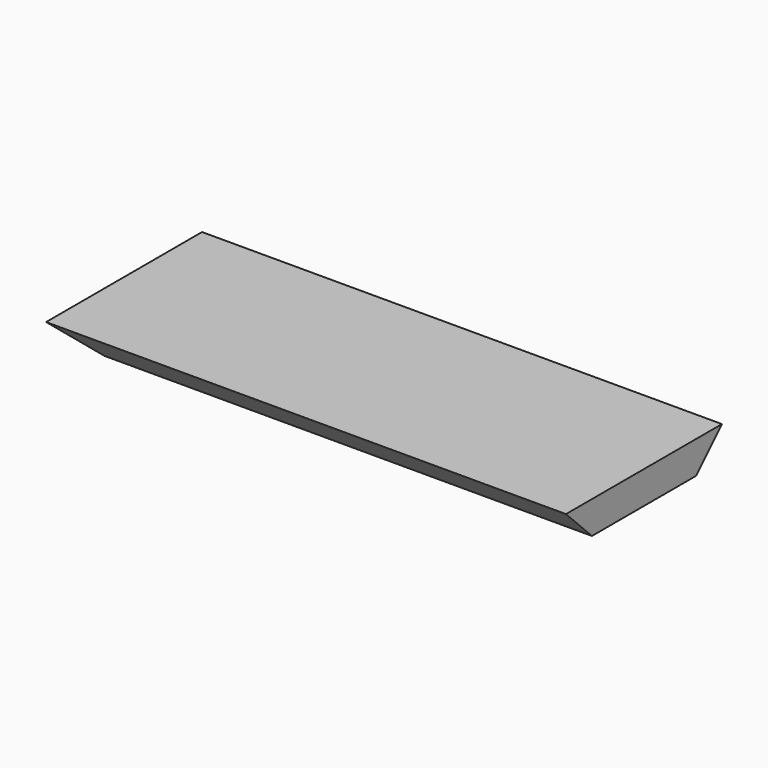
from build123d import *

# Parameters (mm, degrees)
F0_W     = 400
F0_H     = 150
F1_DEPTH = 12.5
F2_SIZE  = 24.99999


# Not quite as in the source:
# - a fillet or chamfer is up to 0.001 mm smaller than in the source, because OpenCascade refuses the exact size


with BuildPart() as f1:
    # F0 (on Top) → F1 (new body, symmetric)
    with BuildSketch(Plane.XY):
        Rectangle(F0_W, F0_H)
    extrude(amount=F1_DEPTH, both=True)

    # F2 (size 25 in the source; OpenCascade refuses exactly that, so slightly less here)
    f2_edges = [f1.edges().sort_by_distance(p)[0] for p in [
        (0, 75, -12.5),
        (-200, 0, -12.5),
        (0, -75, -12.5),
    ]]
    chamfer(f2_edges, length=F2_SIZE)


solid = f1.part
